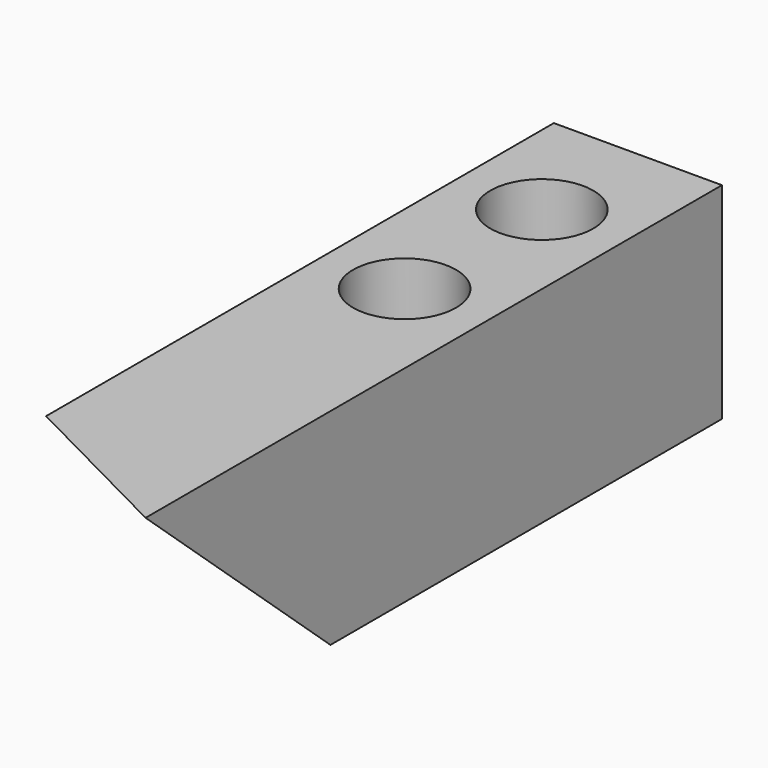
from build123d import *

# Parameters (mm, degrees)
F1_DEPTH = 6
F2_SIZE  = 5.99999
F3_W     = 4.9
F3_H     = 9
F3_R     = 1.5
F4_DEPTH = 6


# Not quite as in the source:
# - a fillet or chamfer is up to 0.001 mm smaller than in the source, because OpenCascade refuses the exact size


with BuildPart() as f1:
    # F0 (on Top) → F1 (new body)
    with BuildSketch(Plane.XY):
        Polygon((-367.6438903809, 71.5354757011), (-372.5438903809, 71.5354757011), (-372.5438903809, 44.0354757011), (-367.6438903809, 41.5354757011), align=None)
    extrude(amount=F1_DEPTH)

    # F2 (size 6 in the source; OpenCascade refuses exactly that, so slightly less here)
    f2_edges = [f1.edges().sort_by_distance(p)[0] for p in [
        (-370.09389, 42.785476, 0),
    ]]
    chamfer(f2_edges, length=F2_SIZE)

    # F3 (on face) → F4 (cut, through all)
    with BuildSketch(Plane.XY.offset(6)):
        with Locations((-370.0938903809, 67.0354757011)):
            Rectangle(F3_W, F3_H)
        with Locations((-370.0938903809, 59.0354757011)):
            Circle(F3_R)
        with Locations((-370.0938903809, 54.0354757011)):
            Circle(F3_R)
    extrude(amount=-F4_DEPTH, mode=Mode.SUBTRACT)


solid = f1.part
